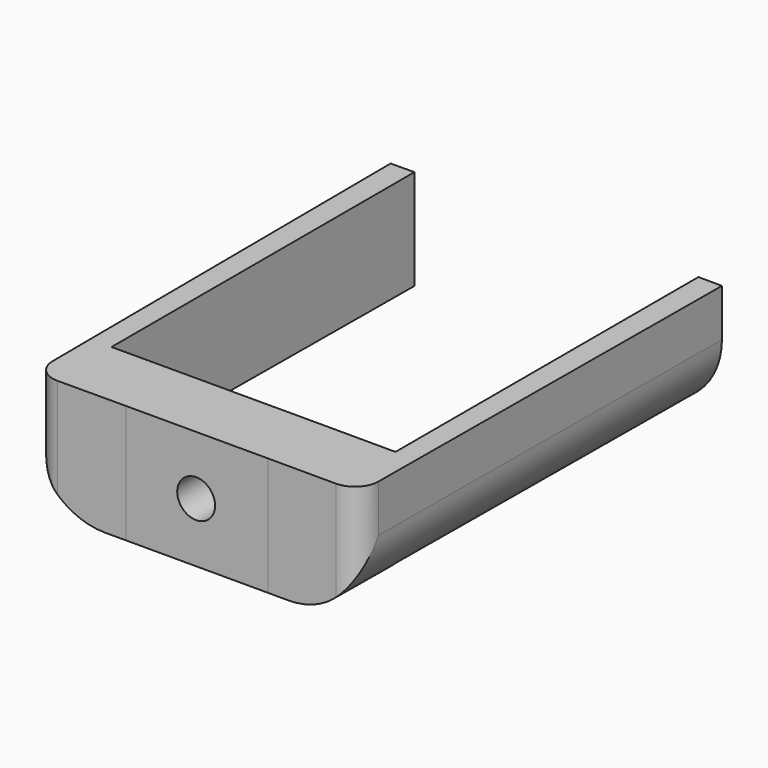
from build123d import *

# Parameters (mm, degrees)
F1_DEPTH    = 25
F2_R        = 4
F3_DEPTH    = 17.8
F4_DEPTH    = 25
F5_T1_DEPTH = 165
F6_T1_DEPTH = 165


# Not quite as in the source:
# - a fillet or chamfer that OpenCascade refuses, or shapes differently, is made with other operations: its cross-section is extruded or revolved along the edge and cut away or added


with BuildPart() as f1:
    # F0 (on Top) → F1 (new body)
    with BuildSketch(Plane.XY):
        with BuildLine():
            ThreePointArc((4.8683269703, 74.3350517786), (8.3924837429, 75.788177233), (9.8682237508, 79.3029241619))
            Line((9.8682237508, 79.3029241619), (10.446520851, 169.3010662119))
            Line((10.446520851, 169.3010662119), (5.4466240705, 169.3331938286))
            Line((5.4466240705, 169.3331938286), (5.4466240705, 89.3331938286))
            Line((5.4466240705, 89.3331938286), (-9.5533759295, 89.3702277541))
            Line((-9.5533759295, 89.3702277541), (-54.5533759295, 89.3331938286))
            Line((-54.5533759295, 89.3331938286), (-54.5533759295, 169.3331938286))
            Line((-54.5533759295, 169.3331938286), (-59.5532727101, 169.3010662119))
            Line((-59.5532727101, 169.3010662119), (-58.9749756099, 79.3029241619))
            ThreePointArc((-58.9749756099, 79.3029241619), (-57.499235602, 75.788177233), (-53.9750788293, 74.3350517786))
            Line((-53.9750788293, 74.3350517786), (-39.5533759295, 74.3702277541))
            Line((-39.5533759295, 74.3702277541), (-9.5533759295, 74.3702277541))
            Line((-9.5533759295, 74.3702277541), (4.8683269703, 74.3350517786))
        make_face()
    extrude(amount=F1_DEPTH)

    # F2 (on face) → F3 (cut)
    with BuildSketch(Plane(origin=(-0.1816306533, 74.4662593781, 0), x_dir=(0.9999970254, 0.0024390927, 0), z_dir=(0.0024390927, -0.9999970254, 0))):
        with Locations((-24.5160218328, 12.5830201432)):
            Circle(F2_R)
    extrude(amount=-F3_DEPTH, mode=Mode.SUBTRACT)

    # F4 (cut): a face of the model
    f4_faces = [f1.faces().sort_by_distance(p)[0] for p in [
        (-24.697579561, 74.4064625271, 12.5830201432),
    ]]
    extrude(f4_faces, amount=-F4_DEPTH, mode=Mode.SUBTRACT)

    # F5: fillet of radius 15 on 1 edges, made by hand

    # F5_s2 → F5_t1 (cut)
    with BuildSketch(Plane(origin=(0.2690025781, 41.8638312931, 0), x_dir=(0, 0, 1), z_dir=(0.0064255233, 0.9999793561, 0))):
        with BuildLine():
            ThreePointArc((0, -5.6415427574), (4.3933982822, 4.9650589604), (15, 9.3584572426))
            Line((15, 9.3584572426), (0, 9.3584572426))
            Line((0, 9.3584572426), (0, -5.6415427574))
        make_face()
    extrude(amount=F5_T1_DEPTH, mode=Mode.SUBTRACT)

    # F6: fillet of radius 15 on 1 edges, made by hand

    # F6_s2 → F6_t1 (cut)
    with BuildSketch(Plane(origin=(-1.3312414161, 207.1759551176, 0), x_dir=(0, 0, 1), z_dir=(0.0064255233, -0.9999793561, 0))):
        with BuildLine():
            ThreePointArc((0, 43.4641953473), (4.3933982822, 54.0707970651), (15, 58.4641953473))
            Line((15, 58.4641953473), (0, 58.4641953473))
            Line((0, 58.4641953473), (0, 43.4641953473))
        make_face()
    extrude(amount=F6_T1_DEPTH, mode=Mode.SUBTRACT)


solid = f1.part
